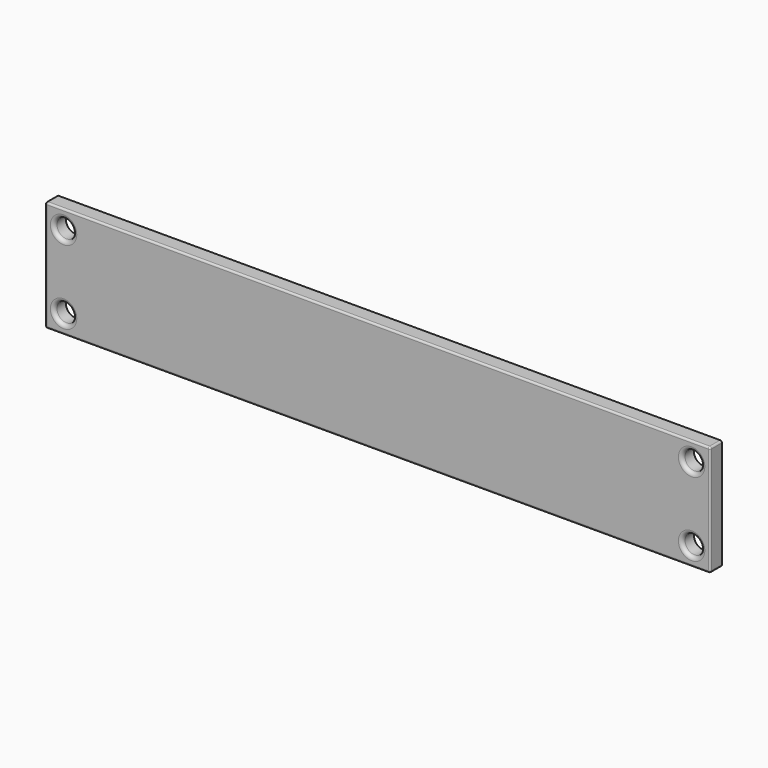
from build123d import *

# Parameters (mm, degrees)
F0_W         = 180
F0_H         = 30
F0_R         = 2.5751263091
F1_DEPTH     = 4
F2_R         = 1
F3_R         = 0.5
F4_TEXT_SIZE = 6.5986184143
F5_DEPTH     = 1


# Not quite as in the source:
# - a feature names something its author has since deleted; it is built from what else it names
# - Text() gives the source's letters only with a copy of the font that has no kerning and outlines rounded to 1/6400 em; it was checked with that copy


with BuildPart() as f1:
    # F0 (on Front) → F1 (new body)
    with BuildSketch(Plane.XZ):
        Rectangle(F0_W, F0_H)
        with Locations((-85, -10)):
            Circle(F0_R, mode=Mode.SUBTRACT)
        with Locations((85, -10)):
            Circle(F0_R, mode=Mode.SUBTRACT)
        with Locations((-85, 10)):
            Circle(F0_R, mode=Mode.SUBTRACT)
        with Locations((85, 10)):
            Circle(F0_R, mode=Mode.SUBTRACT)
    extrude(amount=F1_DEPTH)

    # F2
    f2_edges = [f1.edges().sort_by_distance(p)[0] for p in [
        (-87.575126, -4, 10),
        (-87.575126, -4, -10),
        (82.424874, -4, 10),
        (82.424874, -4, -10),
    ]]
    fillet(f2_edges, radius=F2_R)

    # F3
    f3_edges = [f1.edges().sort_by_distance(p)[0] for p in [
        (0, -4, 15),
        (-90, -4, 0),
        (0, -4, -15),
        (90, -4, 0),
        (-90, -2, 15),
        (-90, -2, -15),
        (90, -2, 15),
        (90, -2, -15),
    ]]
    fillet(f3_edges, radius=F3_R)

    # F4 (on face) → F5 (join)
    with BuildSketch(Plane(origin=(0, 0, 0), x_dir=(-1, 0, 0), z_dir=(0, 1, 0))):
        with Locations((-69.911214523, -0.7829741126)):
            Text('New Berea FP Body', F4_TEXT_SIZE, font='Open Sans', text_align=(TextAlign.LEFT, TextAlign.BOTTOM))
    extrude(amount=F5_DEPTH)

    # F6: F1 across plane


with BuildPart() as f1_1:
    add(f1.part)
    add(f1.part.mirror(Plane.YZ))


solid = f1_1.part
